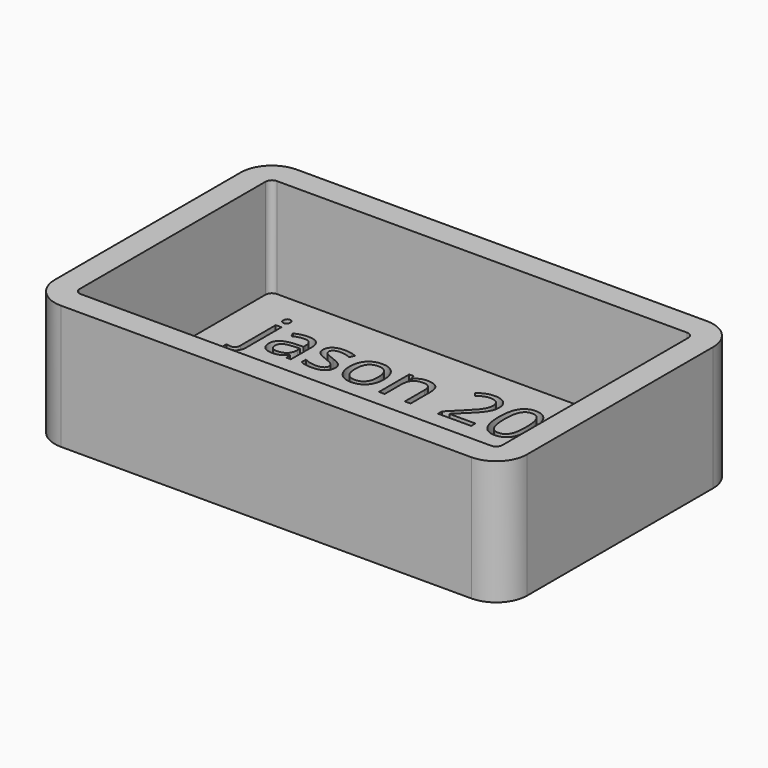
from build123d import *

# Parameters (mm, degrees)
F1_DEPTH     = 25.4
F2_T         = -5.08
F4_START     = 2.54
F3_TEXT_SIZE = 14.4231249578
F4_DEPTH     = 23.622


# Not quite as in the source:
# - Text() gives the source's letters only with a copy of the font that has no kerning and outlines rounded to 1/6400 em; it was checked with that copy


with BuildPart() as f1:
    # F0 (on Top) → F1 (new body)
    with BuildSketch(Plane.XY):
        with BuildLine():
            Line((38.2904044352, 28.9330996206), (-45.5295955648, 28.9330996206))
            ThreePointArc((-45.5295955648, 28.9330996206), (-50.0197236253, 27.0732276811), (-51.8795955648, 22.5830996206))
            Line((-51.8795955648, 22.5830996206), (-51.8795955648, -24.9149003794))
            ThreePointArc((-51.8795955648, -24.9149003794), (-50.0197236253, -29.40502844), (-45.5295955648, -31.2649003794))
            Line((-45.5295955648, -31.2649003794), (38.2904044352, -31.2649003794))
            ThreePointArc((38.2904044352, -31.2649003794), (42.7805324958, -29.40502844), (44.6404044352, -24.9149003794))
            Line((44.6404044352, -24.9149003794), (44.6404044352, 22.5830996206))
            ThreePointArc((44.6404044352, 22.5830996206), (42.7805324958, 27.0732276811), (38.2904044352, 28.9330996206))
        make_face()
    extrude(amount=F1_DEPTH)

    # F2
    f2_openings = [f1.faces().sort_by_distance(p)[0] for p in [
        (-3.619596, -1.1659, 25.4),
    ]]
    offset(amount=F2_T, openings=f2_openings)

    # F3 (on Top) → F4 (cut)
    with BuildSketch(Plane.XY.offset(F4_START)):
        with Locations((-40.1916243136, 7.6384730637)):
            Text('jason 2016', F3_TEXT_SIZE, font='Open Sans', text_align=(TextAlign.LEFT, TextAlign.BOTTOM))
    extrude(amount=F4_DEPTH, mode=Mode.SUBTRACT)


solid = f1.part
